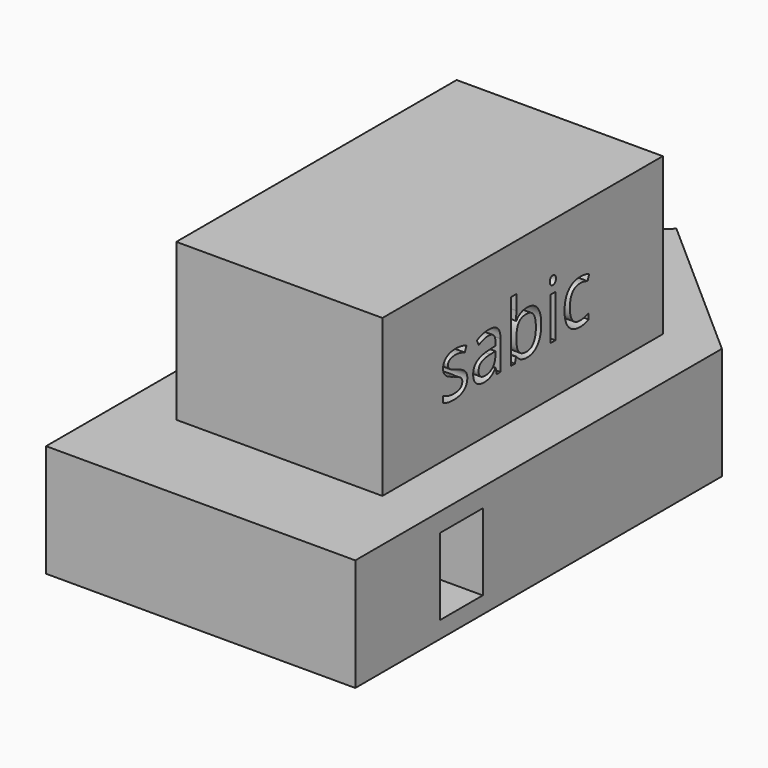
from build123d import *

# Parameters (mm, degrees)
F2_DEPTH     = 27.686
F1_W         = 50.8
F1_H         = 86.36
F3_DEPTH     = 66.294
F6_TEXT_SIZE = 19.6529966262
F7_DEPTH     = 195.326
F8_W         = 13.1155252457
F8_H         = 18.8981262036
F9_DEPTH     = 59.436


# Not quite as in the source:
# - the program builds the solid bodies; features that only make, move or delete a surface that nothing else refers to are left out
# - Text() gives the source's letters only with a copy of the font that has no kerning and outlines rounded to 1/6400 em; it was checked with that copy


with BuildPart() as f2:
    # F0 (on Top) → F2 (new body)
    with BuildSketch(Plane.XY):
        Polygon((38.1, 40.4423935101), (0, 74.0485535808), (-38.1, 40.0516283519), (-38.1, -72.4899148995), (38.1, -72.4899148995), align=None)
    extrude(amount=F2_DEPTH)

    # F1 (on Top) → F3 (join)
    with BuildSketch(Plane.XY):
        with Locations((0, -5.08)):
            Rectangle(F1_W, F1_H)
    extrude(amount=F3_DEPTH)

    # F6 (on face) → F7 (cut)
    with BuildSketch(Plane.YZ.offset(25.4)):
        with Locations((-30.5893085897, 39.7833287716)):
            Text('sabic', F6_TEXT_SIZE, font='Open Sans', text_align=(TextAlign.LEFT, TextAlign.BOTTOM))
    extrude(amount=-F7_DEPTH, mode=Mode.SUBTRACT)

    # F8 (on face) → F9 (cut)
    with BuildSketch(Plane.YZ.offset(38.1)):
        with Locations((-39.7799983621, 13.5783979204)):
            Rectangle(F8_W, F8_H)
    extrude(amount=-F9_DEPTH, mode=Mode.SUBTRACT)


solid = f2.part
